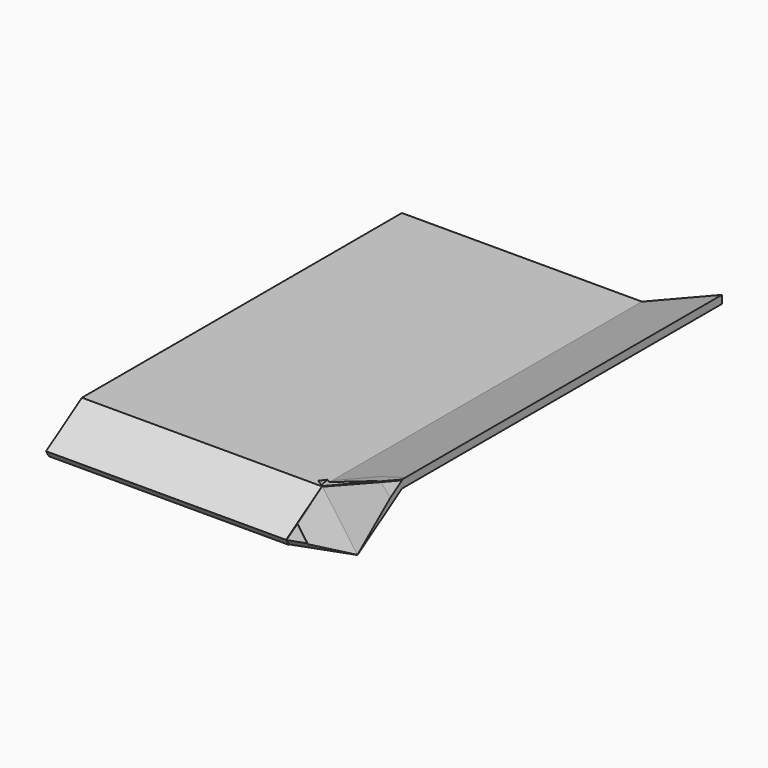
from build123d import *

# Parameters (mm, degrees)
F0_W      = 150
F0_H      = 250
F1_DEPTH  = 5
F3_DEPTH  = 150
F5_DEPTH  = 250
F7_W      = 58.9762479067
F7_H      = 46.3181659579
F8_DEPTH  = 3.61943
F9_W      = 66.3050051284
F9_H      = 23.7932279706
F10_DEPTH = 25
F11_W     = 9.7743958235
F11_H     = 36.3947637379
F12_DEPTH = 25
F13_W     = 91.9819101691
F13_H     = 53.4567786381
F14_DEPTH = 25
F17_DEPTH = 42.79442
F18_DEPTH = 37.25584


with BuildPart() as f1:
    # F0 (on Top) → F1 (new body)
    with BuildSketch(Plane.XY):
        with Locations((75, 125)):
            Rectangle(F0_W, F0_H)
    extrude(amount=F1_DEPTH)

    # F2 (on Right) → F3 (join)
    with BuildSketch(Plane.YZ):
        Polygon((-25.8566159755, -16.7061649263), (0, 0), (0, 5), (-27.978492185, -13.0771259965), align=None)
    extrude(amount=F3_DEPTH)

    # F4 (on Front) → F5 (join)
    with BuildSketch(Plane.XZ):
        Polygon((150, 5), (150, 0), (200, 20), (200, 25), align=None)
    extrude(amount=-F5_DEPTH)

    # F7 (on 3pt) → F8 (join)
    with BuildSketch(Plane(origin=(15.2143755699, 24.5753222078, -38.0359389247), x_dir=(0.9479297598, -0.1728350436, 0.2675018096), z_dir=(-0.3184794663, -0.5144302811, 0.7961986658))):
        with Locations((171.1452230811, -7.3043461889)):
            Rectangle(F7_W, F7_H)
    extrude(amount=F8_DEPTH)

    # F9 (on face) → F10 (cut)
    with BuildSketch(Plane(origin=(18.9655172414, 0, -47.4137931034), x_dir=(0.9284766909, 0, 0.3713906764), z_dir=(-0.3713906764, 0, 0.9284766909))):
        with Locations((174.2809595788, 11.8966139853)):
            Rectangle(F9_W, F9_H)
    extrude(amount=F10_DEPTH, mode=Mode.SUBTRACT)

    # F11 (on face) → F12 (cut)
    with BuildSketch(Plane.XY.offset(5)):
        with Locations((145.1128020883, 18.197381869)):
            Rectangle(F11_W, F11_H)
    extrude(amount=F12_DEPTH, mode=Mode.SUBTRACT)

    # F13 (on face) → F14 (cut)
    with BuildSketch(Plane.YZ.offset(200)):
        with Locations((-13.2915489376, 13.6362598278)):
            Rectangle(F13_W, F13_H)
    extrude(amount=F14_DEPTH, mode=Mode.SUBTRACT)

    # F16 (on face) → F17 (cut)
    with BuildSketch(Plane(origin=(121.6211489037, -89.4544048238, -10.2533341545), x_dir=(0.5890555913, 0.8065651439, -0.0496606377), z_dir=(0.8037140341, -0.5911452179, -0.0677575293))):
        Polygon((66.8091401458, 0), (89.8736044765, 14.5051842555), (116.4209321141, 42.6778681576), align=None)
    extrude(amount=F17_DEPTH, mode=Mode.SUBTRACT)

    # F18 (cut): a face of the model
    f18_faces = [f1.faces().sort_by_distance(p)[0] for p in [
        (175.9683447832, -17.0287264276, 2.5203105636),
    ]]
    extrude(f18_faces, amount=-F18_DEPTH, mode=Mode.SUBTRACT)


solid = f1.part
